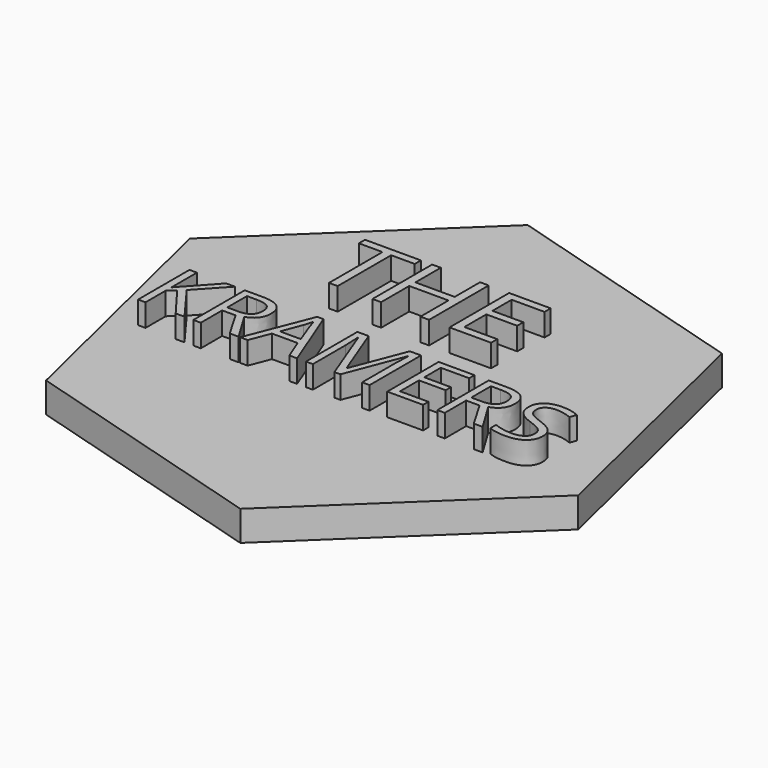
from build123d import *

# Parameters (mm, degrees)
F1_DEPTH       = 5.08
F2_TEXT_SIZE   = 17.6388888889
F2_TEXT_SIZE_2 = 15.2146422629
F3_DEPTH       = 3.81


# Not quite as in the source:
# - Text() gives the source's letters only with a copy of the font that has no kerning and outlines rounded to 1/6400 em; it was checked with that copy


with BuildPart() as f1:
    # F0 (on Top) → F1 (new body)
    with BuildSketch(Plane.XY):
        Polygon((-42.9316082231, 12.6388993647), (-32.4114120372, -30.8604136642), (10.5201961859, -43.4993130289), (42.9316082231, -12.6388993647), (32.4114120372, 30.8604136642), (-10.5201961859, 43.4993130289), align=None)
    extrude(amount=F1_DEPTH)

    # F2 (on face) → F3 (join)
    with BuildSketch(Plane.XY.offset(5.08)):
        with Locations((-20.2379709594, 8.5055471433)):
            Text('THE', F2_TEXT_SIZE, font='Open Sans', text_align=(TextAlign.LEFT, TextAlign.BOTTOM))
        with Locations((-34.29, -10.9545424293)):
            Text('KRAMERS', F2_TEXT_SIZE_2, font='Open Sans', text_align=(TextAlign.LEFT, TextAlign.BOTTOM))
    extrude(amount=F3_DEPTH)


solid = f1.part
